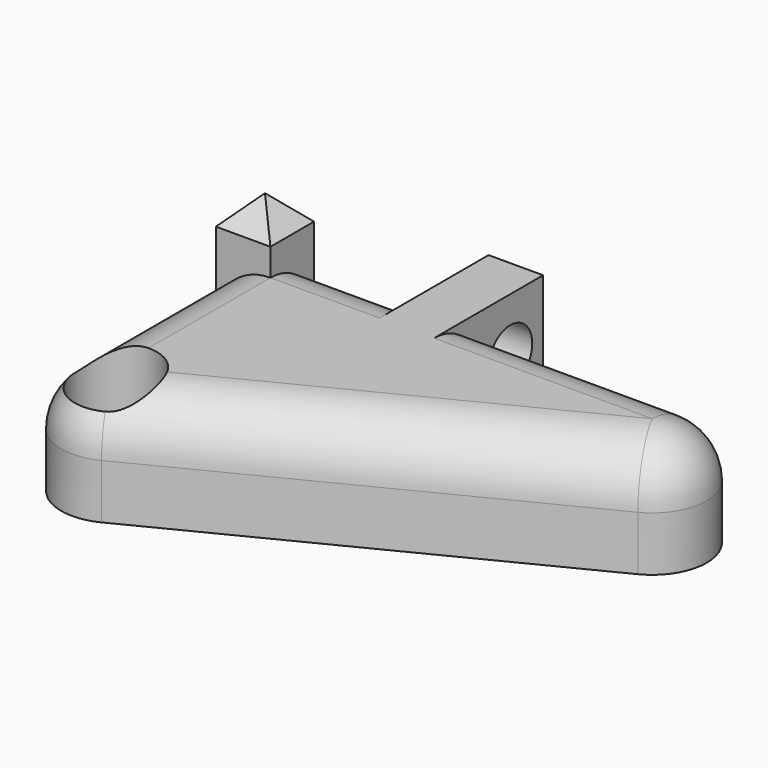
from build123d import *

# Parameters (mm, degrees)
F0_W         = 12.7
F0_H         = 12.7
F0_R         = 9.525
F1_DEPTH     = 25.4
F2_DEPTH     = 38.1
F3_SIZE      = 6.34999
F4_T1_DEPTH  = 50.8
F4_T3_DEPTH  = 99.6409143921
F4_T5_DEPTH  = 25.4
F4_T7_DEPTH  = 45.0011313289
F4_T10_ANGLE = 153.1514920802
F4_T12_ANGLE = 116.8485079198
F5_R         = 6.35
F6_DEPTH     = 50.8010001


# Not quite as in the source:
# - a fillet or chamfer that OpenCascade refuses, or shapes differently, is made with other operations: its cross-section is extruded or revolved along the edge and cut away or added
# - a fillet or chamfer is up to 0.001 mm smaller than in the source, because OpenCascade refuses the exact size


with BuildPart() as f1:
    # F0 (on Top) → F1 (new body)
    with BuildSketch(Plane.XY):
        with Locations((-38.2198102176, 35.4162262917)):
            Rectangle(F0_W, F0_H)
        with BuildLine():
            Line((-6.4698102176, 41.7662262917), (-31.8698102176, 41.7662262917))
            Line((-31.8698102176, 41.7662262917), (-31.8698102176, 29.0662262917))
            Line((-31.8698102176, 29.0662262917), (-44.5698102176, 29.0662262917))
            Line((-44.5698102176, 29.0662262917), (-44.5698102176, -15.9349050373))
            ThreePointArc((-44.5698102176, -15.9349050373), (-31.8698102176, -3.2349050373), (-19.1698102176, -15.9349050373))
            ThreePointArc((-19.1698102176, -15.9349050373), (-21.0500621459, -22.5849465157), (-26.1340703224, -27.2658929842))
            Line((-26.1340703224, -27.2658929842), (62.7659296776, 17.7352383447))
            ThreePointArc((62.7659296776, 17.7352383447), (69.3831964392, 32.0146540993), (57.0301897824, 41.7662262917))
            Line((57.0301897824, 41.7662262917), (6.2301897824, 41.7662262917))
            Line((6.2301897824, 41.7662262917), (6.2301897824, 60.8162262917))
            Line((6.2301897824, 60.8162262917), (-6.4698102176, 60.8162262917))
            Line((-6.4698102176, 60.8162262917), (-6.4698102176, 41.7662262917))
        make_face()
        with BuildLine():
            ThreePointArc((-19.1698102176, -15.9349050373), (-31.8698102176, -3.2349050373), (-44.5698102176, -15.9349050373))
            ThreePointArc((-44.5698102176, -15.9349050373), (-38.5198516961, -26.754653109), (-26.1340703224, -27.2658929842))
            ThreePointArc((-26.1340703224, -27.2658929842), (-21.0500621459, -22.5849465157), (-19.1698102176, -15.9349050373))
        make_face()
        with Locations((-31.8698102176, -15.9349050373)):
            Circle(F0_R, mode=Mode.SUBTRACT)
    extrude(amount=F1_DEPTH)

    # F0 (on Top) → F2 (join)
    with BuildSketch(Plane.XY):
        with Locations((-38.2198102176, 35.4162262917)):
            Rectangle(F0_W, F0_H)
    extrude(amount=F2_DEPTH)

    # F3 (size 6.35 in the source; OpenCascade refuses exactly that, so slightly less here)
    f3_edges = [f1.edges().sort_by_distance(p)[0] for p in [
        (-38.21981, 29.066226, 38.1),
        (-44.56981, 35.416226, 38.1),
        (-38.21981, 41.766226, 38.1),
        (-31.86981, 35.416226, 38.1),
    ]]
    chamfer(f3_edges, length=F3_SIZE)

    # F4: fillet of radius 12.7 on 6 edges, made by hand

    # F4_s2 → F4_t1 (cut)
    with BuildSketch(Plane.YZ.offset(6.2301897824)):
        with BuildLine():
            ThreePointArc((29.0662262917, 25.4), (38.0464824127, 21.6802561211), (41.7662262917, 12.7))
            Line((41.7662262917, 12.7), (42.0202262917, 12.7))
            Line((42.0202262917, 12.7), (42.0202262917, 25.654))
            Line((42.0202262917, 25.654), (29.0662262917, 25.654))
            Line((29.0662262917, 25.654), (29.0662262917, 25.4))
        make_face()
    extrude(amount=F4_T1_DEPTH, mode=Mode.SUBTRACT)

    # F4_s4 → F4_t3 (cut)
    with BuildSketch(Plane(origin=(-31.7901974435, -16.0921805414, 0), x_dir=(0, 0, 1), z_dir=(0.8922037754, 0.4516330626, 0))):
        with BuildLine():
            ThreePointArc((25.4, -0.1762775595), (21.6802561211, 8.8039785616), (12.7, 12.5237224405))
            Line((12.7, 12.5237224405), (12.7, 12.7777224405))
            Line((12.7, 12.7777224405), (25.654, 12.7777224405))
            Line((25.654, 12.7777224405), (25.654, -0.1762775595))
            Line((25.654, -0.1762775595), (25.4, -0.1762775595))
        make_face()
    extrude(amount=F4_T3_DEPTH, mode=Mode.SUBTRACT)

    # F4_s6 → F4_t5 (cut)
    with BuildSketch(Plane.YZ.offset(-31.8698102176)):
        with BuildLine():
            ThreePointArc((41.7662262917, 12.7), (38.0464824127, 21.6802561211), (29.0662262917, 25.4))
            Line((29.0662262917, 25.4), (29.0662262917, 25.654))
            Line((29.0662262917, 25.654), (42.0202262917, 25.654))
            Line((42.0202262917, 25.654), (42.0202262917, 12.7))
            Line((42.0202262917, 12.7), (41.7662262917, 12.7))
        make_face()
    extrude(amount=F4_T5_DEPTH, mode=Mode.SUBTRACT)

    # F4_s8 → F4_t7 (cut)
    with BuildSketch(Plane.XZ.offset(-29.0662262917)):
        with BuildLine():
            ThreePointArc((-44.5698102176, 12.7), (-40.8500663387, 21.6802561211), (-31.8698102176, 25.4))
            Line((-31.8698102176, 25.4), (-31.8698102176, 25.654))
            Line((-31.8698102176, 25.654), (-44.8238102176, 25.654))
            Line((-44.8238102176, 25.654), (-44.8238102176, 12.7))
            Line((-44.8238102176, 12.7), (-44.5698102176, 12.7))
        make_face()
    extrude(amount=F4_T7_DEPTH, mode=Mode.SUBTRACT)

    # F4_s9 → F4_t10 (revolve, cut)
    with BuildSketch(Plane(origin=(57.1098025565, 28.9089507875, 0), x_dir=(0, 0, 1), z_dir=(-0.8922037754, -0.4516330626, 0))):
        with BuildLine():
            ThreePointArc((25.4, 0.1762775595), (21.6802561211, -8.8039785616), (12.7, -12.5237224405))
            Line((12.7, -12.5237224405), (12.7, -12.7777224405))
            Line((12.7, -12.7777224405), (25.654, -12.7777224405))
            Line((25.654, -12.7777224405), (25.654, 0.1762775595))
            Line((25.654, 0.1762775595), (25.4, 0.1762775595))
        make_face()
    revolve(axis=Axis((57.0301897824, 29.0662262917, 25.4), (0, 0, 1)), revolution_arc=F4_T10_ANGLE, mode=Mode.SUBTRACT)

    # F4_s11 → F4_t12 (revolve, cut)
    with BuildSketch(Plane.XZ.offset(15.9349050373)):
        with BuildLine():
            ThreePointArc((-44.5698102176, 12.7), (-40.8500663387, 21.6802561211), (-31.8698102176, 25.4))
            Line((-31.8698102176, 25.4), (-31.8698102176, 25.654))
            Line((-31.8698102176, 25.654), (-44.8238102176, 25.654))
            Line((-44.8238102176, 25.654), (-44.8238102176, 12.7))
            Line((-44.8238102176, 12.7), (-44.5698102176, 12.7))
        make_face()
    revolve(axis=Axis((-31.8698102176, -15.9349050373, 25.4), (0, 0, 1)), revolution_arc=F4_T12_ANGLE, mode=Mode.SUBTRACT)

    # F5 (on face) → F6 (cut, through all)
    with BuildSketch(Plane.YZ.offset(6.2301897824)):
        with Locations((51.2912262917, 12.7)):
            Circle(F5_R)
    extrude(amount=-F6_DEPTH, mode=Mode.SUBTRACT)


solid = f1.part
